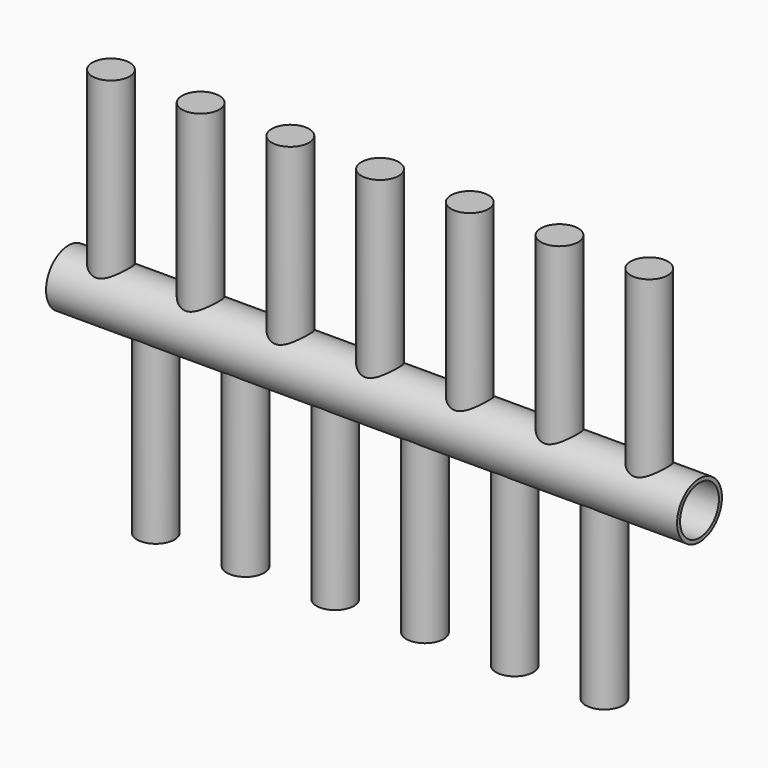
from build123d import *

# Parameters (mm, degrees)
F0_R     = 9.525
F0_R_2   = 8.255
F1_DEPTH = 214.376
F3_DEPTH = 66.802
F4_DEPTH = 66.802


with BuildPart() as f1:
    # F0 (on Right) → F1 (new body)
    with BuildSketch(Plane.YZ):
        Circle(F0_R)
        Circle(F0_R_2, mode=Mode.SUBTRACT)
    extrude(amount=F1_DEPTH)


with BuildPart() as f3:
    # F2 (on Top) → F3 (new body)
    with BuildSketch(Plane.XY):
        with BuildLine():
            ThreePointArc((20.7733392388, 0), (14.4233392388, 6.35), (8.0733392388, 0))
            Line((8.0733392388, 0), (14.4233392388, 0))
            Line((14.4233392388, 0), (20.7733392388, 0))
        make_face()
        with BuildLine():
            Line((14.4233392388, 0), (8.0733392388, 0))
            ThreePointArc((8.0733392388, 0), (14.4233392388, -6.35), (20.7733392388, 0))
            Line((20.7733392388, 0), (14.4233392388, 0))
        make_face()
    extrude(amount=F3_DEPTH)


with BuildPart() as f3b:
    # F2 (on Top) → F3, piece 2 (new body)
    with BuildSketch(Plane.XY):
        with BuildLine():
            ThreePointArc((203.6533392388, 0), (197.3033392388, 6.35), (190.9533392388, 0))
            Line((190.9533392388, 0), (198.5922306776, 0))
            Line((198.5922306776, 0), (203.6533392388, 0))
        make_face()
        with BuildLine():
            Line((198.5922306776, 0), (190.9533392388, 0))
            ThreePointArc((190.9533392388, 0), (197.3033392388, -6.35), (203.6533392388, 0))
            Line((203.6533392388, 0), (198.5922306776, 0))
        make_face()
    extrude(amount=F3_DEPTH)


with BuildPart() as f3c:
    # F2 (on Top) → F3, piece 3 (new body)
    with BuildSketch(Plane.XY):
        with BuildLine():
            ThreePointArc((173.1733392388, 0), (166.8233392388, 6.35), (160.4733392388, 0))
            Line((160.4733392388, 0), (173.1733392388, 0))
        make_face()
        with BuildLine():
            Line((173.1733392388, 0), (160.4733392388, 0))
            ThreePointArc((160.4733392388, 0), (166.8233392388, -6.35), (173.1733392388, 0))
        make_face()
    extrude(amount=F3_DEPTH)


with BuildPart() as f3d:
    # F2 (on Top) → F3, piece 4 (new body)
    with BuildSketch(Plane.XY):
        with BuildLine():
            ThreePointArc((142.6933392388, 0), (136.3433392388, 6.35), (129.9933392388, 0))
            Line((129.9933392388, 0), (142.6933392388, 0))
        make_face()
        with BuildLine():
            Line((142.6933392388, 0), (129.9933392388, 0))
            ThreePointArc((129.9933392388, 0), (136.3433392388, -6.35), (142.6933392388, 0))
        make_face()
    extrude(amount=F3_DEPTH)


with BuildPart() as f3e:
    # F2 (on Top) → F3, piece 5 (new body)
    with BuildSketch(Plane.XY):
        with BuildLine():
            ThreePointArc((112.2133392388, 0), (105.8633392388, 6.35), (99.5133392388, 0))
            Line((99.5133392388, 0), (112.2133392388, 0))
        make_face()
        with BuildLine():
            Line((112.2133392388, 0), (99.5133392388, 0))
            ThreePointArc((99.5133392388, 0), (105.8633392388, -6.35), (112.2133392388, 0))
        make_face()
    extrude(amount=F3_DEPTH)


with BuildPart() as f3f:
    # F2 (on Top) → F3, piece 6 (new body)
    with BuildSketch(Plane.XY):
        with BuildLine():
            ThreePointArc((81.7333392388, 0), (75.3833392388, 6.35), (69.0333392388, 0))
            Line((69.0333392388, 0), (81.7333392388, 0))
        make_face()
        with BuildLine():
            Line((81.7333392388, 0), (69.0333392388, 0))
            ThreePointArc((69.0333392388, 0), (75.3833392388, -6.35), (81.7333392388, 0))
        make_face()
    extrude(amount=F3_DEPTH)


with BuildPart() as f3g:
    # F2 (on Top) → F3, piece 7 (new body)
    with BuildSketch(Plane.XY):
        with BuildLine():
            ThreePointArc((51.2533392388, 0), (44.9033392388, 6.35), (38.5533392388, 0))
            Line((38.5533392388, 0), (51.2533392388, 0))
        make_face()
        with BuildLine():
            Line((51.2533392388, 0), (38.5533392388, 0))
            ThreePointArc((38.5533392388, 0), (44.9033392388, -6.35), (51.2533392388, 0))
        make_face()
    extrude(amount=F3_DEPTH)


with BuildPart() as f4:
    # F2 (on Top) → F4 (new body)
    with BuildSketch(Plane.XY):
        with BuildLine():
            Line((36.0133392388, 0), (23.3133392388, 0))
            ThreePointArc((23.3133392388, 0), (29.6633392388, -6.35), (36.0133392388, 0))
        make_face()
        with BuildLine():
            ThreePointArc((36.0133392388, 0), (29.6633392388, 6.35), (23.3133392388, 0))
            Line((23.3133392388, 0), (36.0133392388, 0))
        make_face()
    extrude(amount=-F4_DEPTH)


with BuildPart() as f4b:
    # F2 (on Top) → F4, piece 2 (new body)
    with BuildSketch(Plane.XY):
        with BuildLine():
            ThreePointArc((66.4933392388, 0), (60.1433392388, 6.35), (53.7933392388, 0))
            Line((53.7933392388, 0), (66.4933392388, 0))
        make_face()
        with BuildLine():
            Line((66.4933392388, 0), (53.7933392388, 0))
            ThreePointArc((53.7933392388, 0), (60.1433392388, -6.35), (66.4933392388, 0))
        make_face()
    extrude(amount=-F4_DEPTH)


with BuildPart() as f4c:
    # F2 (on Top) → F4, piece 3 (new body)
    with BuildSketch(Plane.XY):
        with BuildLine():
            ThreePointArc((96.9733392388, 0), (90.6233392388, 6.35), (84.2733392388, 0))
            Line((84.2733392388, 0), (96.9733392388, 0))
        make_face()
        with BuildLine():
            Line((96.9733392388, 0), (84.2733392388, 0))
            ThreePointArc((84.2733392388, 0), (90.6233392388, -6.35), (96.9733392388, 0))
        make_face()
    extrude(amount=-F4_DEPTH)


with BuildPart() as f4d:
    # F2 (on Top) → F4, piece 4 (new body)
    with BuildSketch(Plane.XY):
        with BuildLine():
            ThreePointArc((127.4533392388, 0), (121.1033392388, 6.35), (114.7533392388, 0))
            Line((114.7533392388, 0), (127.4533392388, 0))
        make_face()
        with BuildLine():
            Line((127.4533392388, 0), (114.7533392388, 0))
            ThreePointArc((114.7533392388, 0), (121.1033392388, -6.35), (127.4533392388, 0))
        make_face()
    extrude(amount=-F4_DEPTH)


with BuildPart() as f4e:
    # F2 (on Top) → F4, piece 5 (new body)
    with BuildSketch(Plane.XY):
        with BuildLine():
            ThreePointArc((157.9333392388, 0), (151.5833392388, 6.35), (145.2333392388, 0))
            Line((145.2333392388, 0), (157.9333392388, 0))
        make_face()
        with BuildLine():
            Line((157.9333392388, 0), (145.2333392388, 0))
            ThreePointArc((145.2333392388, 0), (151.5833392388, -6.35), (157.9333392388, 0))
        make_face()
    extrude(amount=-F4_DEPTH)


with BuildPart() as f4f:
    # F2 (on Top) → F4, piece 6 (new body)
    with BuildSketch(Plane.XY):
        with BuildLine():
            ThreePointArc((188.4133392388, 0), (182.0633392388, 6.35), (175.7133392388, 0))
            Line((175.7133392388, 0), (188.4133392388, 0))
        make_face()
        with BuildLine():
            Line((188.4133392388, 0), (175.7133392388, 0))
            ThreePointArc((175.7133392388, 0), (182.0633392388, -6.35), (188.4133392388, 0))
        make_face()
    extrude(amount=-F4_DEPTH)


solid = Compound([f1.part, f3.part, f3b.part, f3c.part, f3d.part, f3e.part, f3f.part, f3g.part, f4.part, f4b.part, f4c.part, f4d.part, f4e.part, f4f.part])
